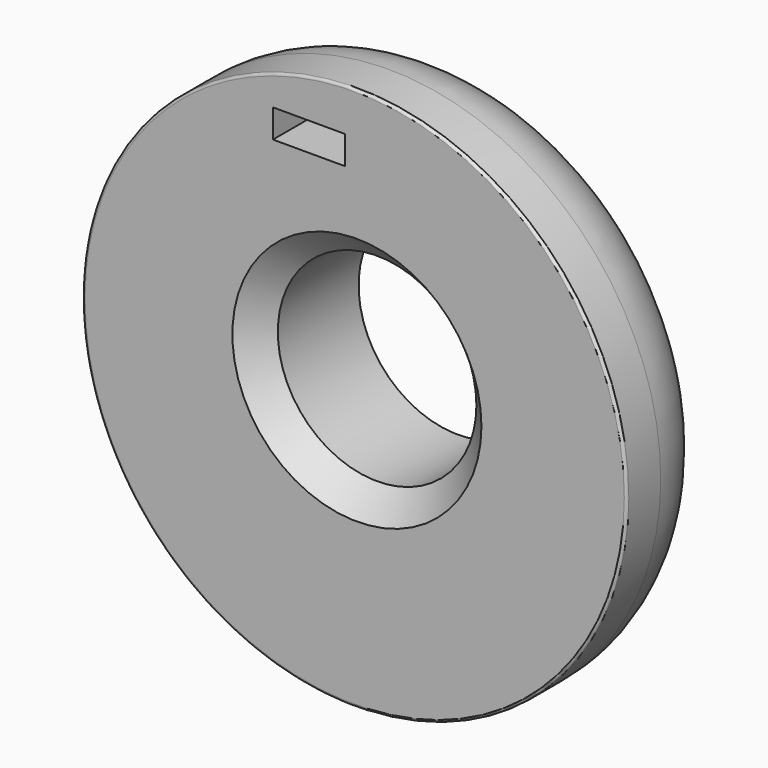
from build123d import *

# Parameters (mm, degrees)
F0_R     = 54.7615085619
F0_R_2   = 19.9782226064
F1_DEPTH = 25.4
F2_W     = 14.4728478044
F2_H     = 5.7084001601
F3_DEPTH = 25.4
F4_R     = 0.508
F5_SIZE  = 5.08


# Not quite as in the source:
# - a fillet or chamfer that OpenCascade refuses, or shapes differently, is made with other operations: its cross-section is extruded or revolved along the edge and cut away or added


with BuildPart() as f1:
    # F0 (on Front) → F1 (new body)
    with BuildSketch(Plane.XZ):
        with Locations((-1.2108273804, -0.5243010819)):
            Circle(F0_R)
        with Locations((-0.7577873766, 2.7753412724)):
            Circle(F0_R_2, mode=Mode.SUBTRACT)
    extrude(amount=F1_DEPTH)

    # F2 (on face) → F3 (cut)
    with BuildSketch(Plane.XZ.offset(25.4)):
        with Locations((-10.4092946276, 42.7569095045)):
            Rectangle(F2_W, F2_H)
    extrude(amount=-F3_DEPTH, mode=Mode.SUBTRACT)

    # F4
    f4_edges = [f1.edges().sort_by_distance(p)[0] for p in [
        (-55.972336, -25.4, -0.524301),
    ]]
    fillet(f4_edges, radius=F4_R)

    # F5
    f5_edges = [f1.edges().sort_by_distance(p)[0] for p in [
        (-20.73601, -25.4, 2.775341),
    ]]
    chamfer(f5_edges, length=F5_SIZE)

    # F6: fillet of radius 16.8651706448 on 1 edges, made by hand

    # F6_s1 → F6_t2 (revolve, cut)
    with BuildSketch(Plane.XY.offset(-0.5243010819)):
        with BuildLine():
            ThreePointArc((53.5506811815, -16.8651706448), (48.6109870655, -4.939694116), (36.6855105367, 0))
            Line((36.6855105367, 0), (53.5506811815, 0))
            Line((53.5506811815, 0), (53.5506811815, -16.8651706448))
        make_face()
    revolve(axis=Axis((-1.2108273804, 0, -0.5243010819), (0, -1, 0)), mode=Mode.SUBTRACT)


solid = f1.part
